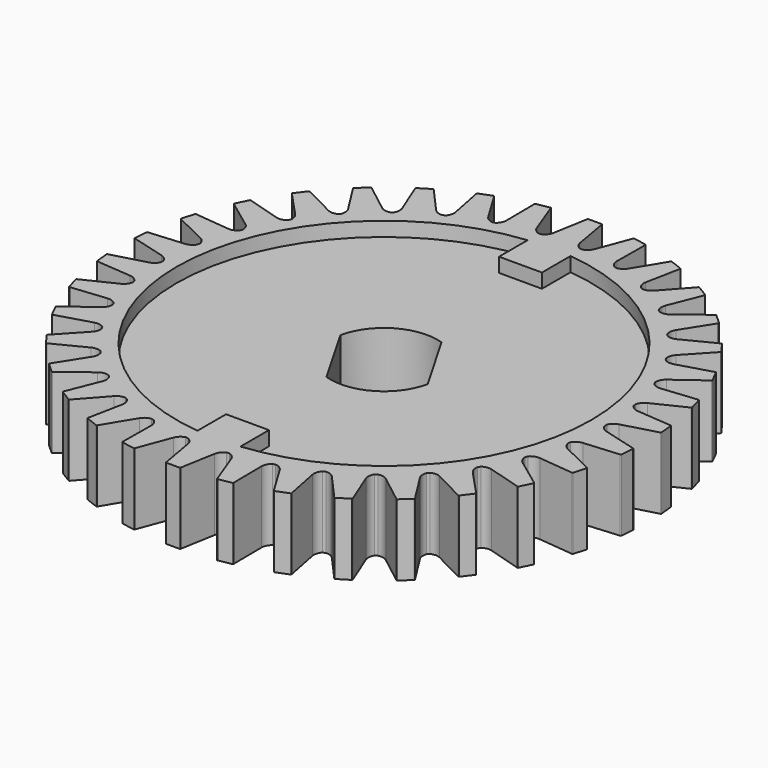
from build123d import *

# Parameters (mm, degrees)
F0_R            = 31
F1_DEPTH        = 10
F3_DEPTH        = 10
F3_COPIES_COUNT = 34
F5_DEPTH        = 2
F7_DEPTH        = 25


# Not quite as in the source:
# - a pattern or mirror of a feature is missing from the dataset's text; its kind, count and spacing are read off the source's solid


with BuildPart() as f1:
    # F0 (on Top) → F1 (new body)
    with BuildSketch(Plane.XY):
        Circle(F0_R)
    extrude(amount=F1_DEPTH)

    # F2 (on face) → F3 (join)
    with BuildSketch(Plane.XY.offset(10)):
        with BuildLine():
            Line((0.9160900369, 36.8852944707), (-0.9160900369, 36.8852944707))
            ThreePointArc((-0.9160900369, 36.8852944707), (-0.9803687979, 36.861898915), (-1.0145708122, 36.8026592885))
            Line((-1.0145708122, 36.8026592885), (-1.8682408883, 31.9612557056))
            ThreePointArc((-1.8682408883, 31.9612557056), (-2.1396172597, 31.3295613228), (-2.6643170715, 30.8852944707))
            ThreePointArc((-2.6643170715, 30.8852944707), (0, 31), (2.6643170715, 30.8852944707))
            ThreePointArc((2.6643170715, 30.8852944707), (2.1396172597, 31.3295613228), (1.8682408883, 31.9612557056))
            Line((1.8682408883, 31.9612557056), (1.0145708122, 36.8026592885))
            ThreePointArc((1.0145708122, 36.8026592885), (0.9803687979, 36.861898915), (0.9160900369, 36.8852944707))
        make_face()
    f3 = extrude(amount=-F3_DEPTH)

    # F3_copies: F3 ×34 about axis
    f3_copies_axis = Axis((0, 0, 0), (0, 0, 1))
    for i in range(1, F3_COPIES_COUNT):
        add(f3.rotate(f3_copies_axis, i * 360 / F3_COPIES_COUNT))

    # F4 (on face) → F5 (cut)
    with BuildSketch(Plane.XY.offset(10)):
        with BuildLine():
            Line((-3, 23.8544972411), (-3, 28.8444102037))
            ThreePointArc((-3, 28.8444102037), (-29, 0), (-3, -28.8444102037))
            Line((-3, -28.8444102037), (-3, -23.8544972411))
            Line((-3, -23.8544972411), (3, -23.8544972411))
            Line((3, -23.8544972411), (3, -28.8444102037))
            ThreePointArc((3, -28.8444102037), (21.5406592285, -19.4164878389), (29, 0))
            ThreePointArc((29, 0), (21.5406592285, 19.4164878389), (3, 28.8444102037))
            Line((3, 28.8444102037), (3, 23.8544972411))
            Line((3, 23.8544972411), (-3, 23.8544972411))
        make_face()
    extrude(amount=-F5_DEPTH, mode=Mode.SUBTRACT)

    # F6 (on face) → F7 (cut)
    with BuildSketch(Plane.XY.offset(8)):
        with BuildLine():
            Line((-7.3412291828, 1.535042047), (-2.3412291828, -7.1252119908))
            ThreePointArc((-2.3412291828, -7.1252119908), (3.75, -6.4951905284), (7.3412291828, -1.535042047))
            Line((7.3412291828, -1.535042047), (2.3412291828, 7.1252119908))
            ThreePointArc((2.3412291828, 7.1252119908), (-3.75, 6.4951905284), (-7.3412291828, 1.535042047))
        make_face()
    extrude(amount=-F7_DEPTH, mode=Mode.SUBTRACT)


solid = f1.part
